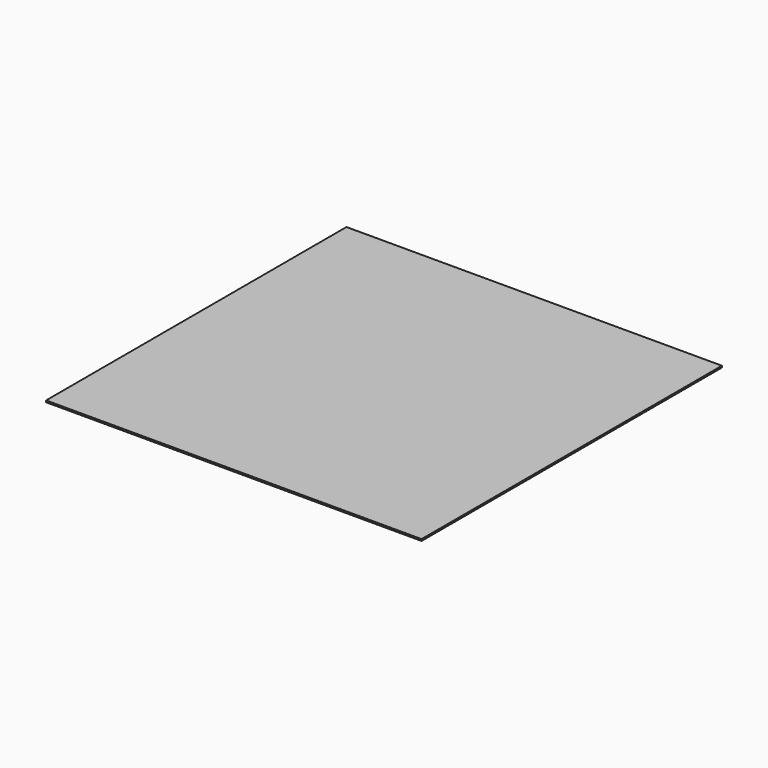
from build123d import *

# Parameters (mm, degrees)
F0_W     = 1000
F0_H     = 1000
F1_DEPTH = 4.5


# Not quite as in the source:
# - a feature names something its author has since deleted; it is built from what else it names


with BuildPart() as f1:
    # F0 (on Top) → F1 (new body)
    with BuildSketch(Plane.XY):
        Rectangle(F0_W, F0_H)
    extrude(amount=F1_DEPTH)


solid = f1.part
